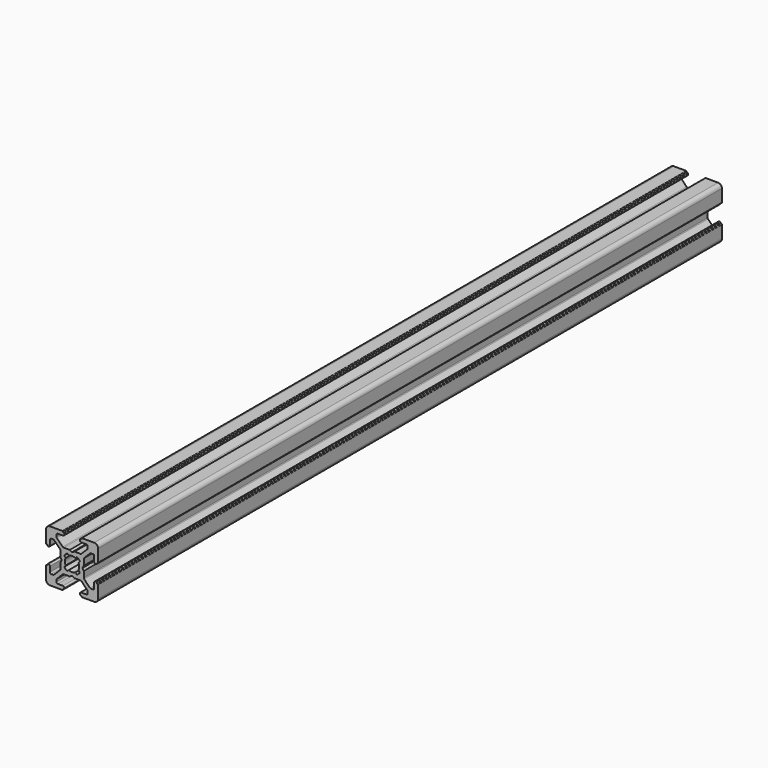
from build123d import *

# Parameters (mm, degrees)
F1_DEPTH = 300


# Not quite as in the source:
# - ends of sketch curves that miss each other by under 0.0002 mm in the source are joined


with BuildPart() as f1:
    # F0 (on Front) → F1 (new body)
    with BuildSketch(Plane.XZ):
        with BuildLine():
            ThreePointArc((-222.93, -209.58), (-222.9885786438, -209.4385786438), (-223.13, -209.38))
            Line((-223.13, -209.38), (-227.88, -209.38))
            ThreePointArc((-227.88, -209.38), (-228.9406601718, -209.8193398282), (-229.38, -210.88))
            Line((-229.38, -210.88), (-229.38, -215.63))
            ThreePointArc((-229.38, -215.63), (-229.3214213562, -215.7714213562), (-229.18, -215.83))
            Line((-229.18, -215.83), (-229.08, -215.83))
            ThreePointArc((-229.08, -215.83), (-228.9385786438, -215.8885786438), (-228.88, -216.03))
            Line((-228.88, -216.03), (-228.88, -216.18))
            ThreePointArc((-228.88, -216.18), (-228.8214213562, -216.3214213562), (-228.68, -216.38))
            Line((-228.68, -216.38), (-228.38, -216.38))
            ThreePointArc((-228.38, -216.38), (-228.0264466094, -216.2335533906), (-227.88, -215.88))
            Line((-227.88, -215.88), (-227.88, -213.88))
            ThreePointArc((-227.88, -213.88), (-227.7335533906, -213.5264466094), (-227.38, -213.38))
            Line((-227.38, -213.38), (-226.647767, -213.38))
            ThreePointArc((-226.647767, -213.38), (-226.4564249572, -213.418060369), (-226.2942131094, -213.5264471094))
            Line((-226.2942131094, -213.5264471094), (-224.026446, -215.794214))
            ThreePointArc((-224.026446, -215.794214), (-223.9180600984, -215.9564256105), (-223.88, -216.147767))
            Line((-223.88, -216.147767), (-223.88, -218.426411))
            ThreePointArc((-223.88, -218.426411), (-223.87318516, -218.4781748285), (-223.8532050606, -218.526411035))
            Line((-223.8532050606, -218.526411035), (-223.41812, -219.28))
            ThreePointArc((-223.41812, -219.28), (-223.391325, -219.38), (-223.4181199394, -219.480000035))
            Line((-223.4181199394, -219.480000035), (-223.853205, -220.233589))
            ThreePointArc((-223.853205, -220.233589), (-223.87318516, -220.2818251715), (-223.88, -220.333589))
            Line((-223.88, -220.333589), (-223.88, -222.612233))
            ThreePointArc((-223.88, -222.612233), (-223.9180600984, -222.8035743895), (-224.0264461094, -222.9657858906))
            Line((-224.0264461094, -222.9657858906), (-226.294213, -225.233553))
            ThreePointArc((-226.294213, -225.233553), (-226.4564249572, -225.341939631), (-226.647767, -225.38))
            Line((-226.647767, -225.38), (-227.38, -225.38))
            ThreePointArc((-227.38, -225.38), (-227.7335533906, -225.2335533906), (-227.88, -224.88))
            Line((-227.88, -224.88), (-227.88, -222.88))
            ThreePointArc((-227.88, -222.88), (-228.0264466094, -222.5264466094), (-228.38, -222.38))
            Line((-228.38, -222.38), (-228.68, -222.38))
            ThreePointArc((-228.68, -222.38), (-228.8214213562, -222.4385786438), (-228.88, -222.58))
            Line((-228.88, -222.58), (-228.88, -222.73))
            ThreePointArc((-228.88, -222.73), (-228.9385786438, -222.8714213562), (-229.08, -222.93))
            Line((-229.08, -222.93), (-229.18, -222.93))
            ThreePointArc((-229.18, -222.93), (-229.3214213562, -222.9885786438), (-229.38, -223.13))
            Line((-229.38, -223.13), (-229.38, -227.88))
            ThreePointArc((-229.38, -227.88), (-228.9406601718, -228.9406601718), (-227.88, -229.38))
            Line((-227.88, -229.38), (-223.13, -229.38))
            ThreePointArc((-223.13, -229.38), (-222.9885786438, -229.3214213562), (-222.93, -229.18))
            Line((-222.93, -229.18), (-222.93, -229.08))
            ThreePointArc((-222.93, -229.08), (-222.8714213562, -228.9385786438), (-222.73, -228.88))
            Line((-222.73, -228.88), (-222.58, -228.88))
            ThreePointArc((-222.58, -228.88), (-222.4385786438, -228.8214213562), (-222.38, -228.68))
            Line((-222.38, -228.68), (-222.38, -228.38))
            ThreePointArc((-222.38, -228.38), (-222.5264466094, -228.0264466094), (-222.88, -227.88))
            Line((-222.88, -227.88), (-224.880001, -227.88))
            ThreePointArc((-224.880001, -227.88), (-225.2335543906, -227.7335533906), (-225.380001, -227.38))
            Line((-225.380001, -227.38), (-225.380001, -226.647767))
            ThreePointArc((-225.380001, -226.647767), (-225.341940631, -226.4564249572), (-225.2335538906, -226.2942131094))
            Line((-225.2335538906, -226.2942131094), (-222.965787, -224.026447))
            ThreePointArc((-222.965787, -224.026447), (-222.8035757162, -223.9180602337), (-222.612234, -223.88))
            Line((-222.612234, -223.88), (-220.33359, -223.88))
            ThreePointArc((-220.33359, -223.88), (-220.2818261715, -223.87318516), (-220.233589965, -223.8532050606))
            Line((-220.233589965, -223.8532050606), (-219.48, -223.41812))
            ThreePointArc((-219.48, -223.41812), (-219.38, -223.391325), (-219.279999965, -223.4181199394))
            Line((-219.279999965, -223.4181199394), (-218.52641, -223.853205))
            ThreePointArc((-218.52641, -223.853205), (-218.4781738285, -223.87318516), (-218.42641, -223.88))
            Line((-218.42641, -223.88), (-216.147766, -223.88))
            ThreePointArc((-216.147766, -223.88), (-215.9564242838, -223.9180602337), (-215.7942126094, -224.0264466094))
            Line((-215.7942126094, -224.0264466094), (-213.526446, -226.294213))
            ThreePointArc((-213.526446, -226.294213), (-213.418059369, -226.4564249572), (-213.379999, -226.647767))
            Line((-213.379999, -226.647767), (-213.379999, -227.38))
            ThreePointArc((-213.379999, -227.38), (-213.5264456094, -227.7335533906), (-213.879999, -227.88))
            Line((-213.879999, -227.88), (-215.88, -227.88))
            ThreePointArc((-215.88, -227.88), (-216.2335533906, -228.0264466094), (-216.38, -228.38))
            Line((-216.38, -228.38), (-216.38, -228.68))
            ThreePointArc((-216.38, -228.68), (-216.3214213562, -228.8214213562), (-216.18, -228.88))
            Line((-216.18, -228.88), (-216.03, -228.88))
            ThreePointArc((-216.03, -228.88), (-215.8885786438, -228.9385786438), (-215.83, -229.08))
            Line((-215.83, -229.08), (-215.83, -229.18))
            ThreePointArc((-215.83, -229.18), (-215.7714213562, -229.3214213562), (-215.63, -229.38))
            Line((-215.63, -229.38), (-210.88, -229.38))
            ThreePointArc((-210.88, -229.38), (-209.8193398282, -228.9406601718), (-209.38, -227.88))
            Line((-209.38, -227.88), (-209.38, -223.13))
            ThreePointArc((-209.38, -223.13), (-209.4385786438, -222.9885786438), (-209.58, -222.93))
            Line((-209.58, -222.93), (-209.68, -222.93))
            ThreePointArc((-209.68, -222.93), (-209.8214213562, -222.8714213562), (-209.88, -222.73))
            Line((-209.88, -222.73), (-209.88, -222.58))
            ThreePointArc((-209.88, -222.58), (-209.9385786438, -222.4385786438), (-210.08, -222.38))
            Line((-210.08, -222.38), (-210.38, -222.38))
            ThreePointArc((-210.38, -222.38), (-210.7335533906, -222.5264466094), (-210.88, -222.88))
            Line((-210.88, -222.88), (-210.88, -224.88))
            ThreePointArc((-210.88, -224.88), (-211.0264466094, -225.2335533906), (-211.38, -225.38))
            Line((-211.38, -225.38), (-212.112233, -225.38))
            ThreePointArc((-212.112233, -225.38), (-212.3035750428, -225.341939631), (-212.4657868906, -225.2335528906))
            Line((-212.4657868906, -225.2335528906), (-214.733554, -222.965786))
            ThreePointArc((-214.733554, -222.965786), (-214.8419399016, -222.8035743895), (-214.88, -222.612233))
            Line((-214.88, -222.612233), (-214.88, -220.333589))
            ThreePointArc((-214.88, -220.333589), (-214.88681484, -220.2818251715), (-214.9067949394, -220.233588965))
            Line((-214.9067949394, -220.233588965), (-215.34188, -219.48))
            ThreePointArc((-215.34188, -219.48), (-215.368675, -219.38), (-215.3418800606, -219.279999965))
            Line((-215.3418800606, -219.279999965), (-214.906795, -218.526411))
            ThreePointArc((-214.906795, -218.526411), (-214.88681484, -218.4781748285), (-214.88, -218.426411))
            Line((-214.88, -218.426411), (-214.88, -216.147767))
            ThreePointArc((-214.88, -216.147767), (-214.8419399016, -215.9564256105), (-214.7335538906, -215.7942141094))
            Line((-214.7335538906, -215.7942141094), (-212.465787, -213.526447))
            ThreePointArc((-212.465787, -213.526447), (-212.3035750428, -213.418060369), (-212.112233, -213.38))
            Line((-212.112233, -213.38), (-211.38, -213.38))
            ThreePointArc((-211.38, -213.38), (-211.0264466094, -213.5264466094), (-210.88, -213.88))
            Line((-210.88, -213.88), (-210.88, -215.88))
            ThreePointArc((-210.88, -215.88), (-210.7335533906, -216.2335533906), (-210.38, -216.38))
            Line((-210.38, -216.38), (-210.08, -216.38))
            ThreePointArc((-210.08, -216.38), (-209.9385786438, -216.3214213562), (-209.88, -216.18))
            Line((-209.88, -216.18), (-209.88, -216.03))
            ThreePointArc((-209.88, -216.03), (-209.8214213562, -215.8885786438), (-209.68, -215.83))
            Line((-209.68, -215.83), (-209.58, -215.83))
            ThreePointArc((-209.58, -215.83), (-209.4385786438, -215.7714213562), (-209.38, -215.63))
            Line((-209.38, -215.63), (-209.38, -210.88))
            ThreePointArc((-209.38, -210.88), (-209.8193398282, -209.8193398282), (-210.88, -209.38))
            Line((-210.88, -209.38), (-215.63, -209.38))
            ThreePointArc((-215.63, -209.38), (-215.7714213562, -209.4385786438), (-215.83, -209.58))
            Line((-215.83, -209.58), (-215.83, -209.68))
            ThreePointArc((-215.83, -209.68), (-215.8885786438, -209.8214213562), (-216.03, -209.88))
            Line((-216.03, -209.88), (-216.18, -209.88))
            ThreePointArc((-216.18, -209.88), (-216.3214213562, -209.9385786438), (-216.38, -210.08))
            Line((-216.38, -210.08), (-216.38, -210.38))
            ThreePointArc((-216.38, -210.38), (-216.2335533906, -210.7335533906), (-215.88, -210.88))
            Line((-215.88, -210.88), (-213.879999, -210.88))
            ThreePointArc((-213.879999, -210.88), (-213.5264456094, -211.0264466094), (-213.379999, -211.38))
            Line((-213.379999, -211.38), (-213.379999, -212.112233))
            ThreePointArc((-213.379999, -212.112233), (-213.418059369, -212.3035750428), (-213.5264461094, -212.4657868906))
            Line((-213.5264461094, -212.4657868906), (-215.794213, -214.733553))
            ThreePointArc((-215.794213, -214.733553), (-215.9564242838, -214.8419397663), (-216.147766, -214.88))
            Line((-216.147766, -214.88), (-218.42641, -214.88))
            ThreePointArc((-218.42641, -214.88), (-218.4781738285, -214.88681484), (-218.526410035, -214.9067949394))
            Line((-218.526410035, -214.9067949394), (-219.28, -215.34188))
            ThreePointArc((-219.28, -215.34188), (-219.38, -215.368675), (-219.480000035, -215.3418800606))
            Line((-219.480000035, -215.3418800606), (-220.23359, -214.906795))
            ThreePointArc((-220.23359, -214.906795), (-220.2818261715, -214.88681484), (-220.33359, -214.88))
            Line((-220.33359, -214.88), (-222.612234, -214.88))
            ThreePointArc((-222.612234, -214.88), (-222.8035757162, -214.8419397663), (-222.9657873906, -214.7335533906))
            Line((-222.9657873906, -214.7335533906), (-225.233554, -212.465787))
            ThreePointArc((-225.233554, -212.465787), (-225.341940631, -212.3035750428), (-225.380001, -212.112233))
            Line((-225.380001, -212.112233), (-225.380001, -211.38))
            ThreePointArc((-225.380001, -211.38), (-225.2335543906, -211.0264466094), (-224.880001, -210.88))
            Line((-224.880001, -210.88), (-222.88, -210.88))
            ThreePointArc((-222.88, -210.88), (-222.5264466094, -210.7335533906), (-222.38, -210.38))
            Line((-222.38, -210.38), (-222.38, -210.08))
            ThreePointArc((-222.38, -210.08), (-222.4385786438, -209.9385786438), (-222.58, -209.88))
            Line((-222.58, -209.88), (-222.73, -209.88))
            ThreePointArc((-222.73, -209.88), (-222.8714213562, -209.8214213562), (-222.93, -209.68))
            Line((-222.93, -209.68), (-222.93, -209.58))
        make_face()
        with BuildLine():
            Line((-221.825295, -218.121815), (-222.372175, -217.470069))
            ThreePointArc((-222.372175, -217.470069), (-221.8917370376, -216.8715897062), (-221.2938948305, -216.3903592648))
            Line((-221.2938948305, -216.3903592648), (-220.638185, -216.934705))
            ThreePointArc((-220.638185, -216.934705), (-219.38, -216.63), (-218.1218147614, -216.9347045362))
            Line((-218.1218147614, -216.9347045362), (-217.466105, -216.390359))
            ThreePointArc((-217.466105, -216.390359), (-216.8682629624, -216.8715897062), (-216.3878252977, -217.47006919))
            Line((-216.3878252977, -217.47006919), (-216.934705, -218.121815))
            ThreePointArc((-216.934705, -218.121815), (-216.63, -219.38), (-216.9347045362, -220.6381852386))
            Line((-216.9347045362, -220.6381852386), (-216.387825, -221.289931))
            ThreePointArc((-216.387825, -221.289931), (-216.8682629624, -221.8884102938), (-217.4661051695, -222.3696407352))
            Line((-217.4661051695, -222.3696407352), (-218.121815, -221.825295))
            ThreePointArc((-218.121815, -221.825295), (-219.38, -222.13), (-220.6381852386, -221.8252954638))
            Line((-220.6381852386, -221.8252954638), (-221.293895, -222.369641))
            ThreePointArc((-221.293895, -222.369641), (-221.8917370376, -221.8884102938), (-222.3721747023, -221.28993081))
            Line((-222.3721747023, -221.28993081), (-221.825295, -220.638185))
            ThreePointArc((-221.825295, -220.638185), (-222.13, -219.38), (-221.825295, -218.121815))
        make_face(mode=Mode.SUBTRACT)
    extrude(amount=F1_DEPTH)


with BuildPart() as f1_1:
    # F3: moved
    add(f1.part.moved(Location((219.38, 0, 219.38))))


solid = f1_1.part
